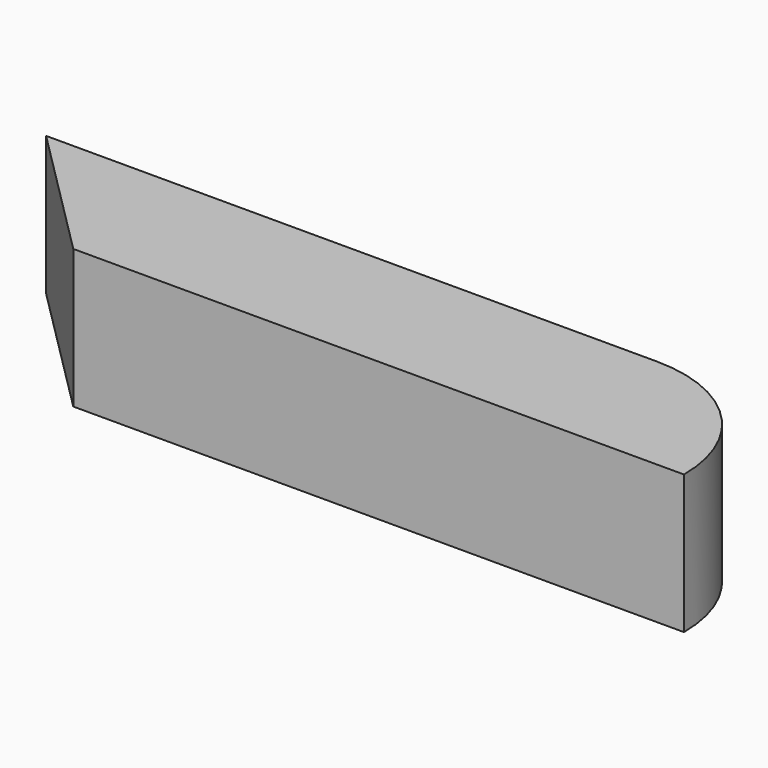
from build123d import *

# Parameters (mm, degrees)
F0_W     = 68.326
F0_H     = 12.446
F1_DEPTH = 12.7
F2_SIZE  = 12.44599
F3_R     = 12.44599
F5_D     = 6.35
F5_DEPTH = 8.89
F5_TIP   = 1.9077324654


# Not quite as in the source:
# - a fillet or chamfer is up to 0.001 mm smaller than in the source, because OpenCascade refuses the exact size


with BuildPart() as f1:
    # F0 (on Top) → F1 (new body)
    with BuildSketch(Plane.XY):
        Rectangle(F0_W, F0_H)
    extrude(amount=F1_DEPTH)

    # F2 (size 12.446 in the source; OpenCascade refuses exactly that, so slightly less here)
    f2_edges = [f1.edges().sort_by_distance(p)[0] for p in [
        (-34.163, -6.223, 6.35),
    ]]
    chamfer(f2_edges, length=F2_SIZE)

    # F3 (radius 12.446 in the source; OpenCascade refuses exactly that, so slightly less here)
    f3_edges = [f1.edges().sort_by_distance(p)[0] for p in [
        (34.163, 6.223, 6.35),
    ]]
    fillet(f3_edges, radius=F3_R)

    # F5
    with Locations(Plane(origin=(0, 0, 0), x_dir=(1, 0, 0), z_dir=(0, 0, -1))):
        with Locations((0, 0)):
            Hole(F5_D / 2, depth=F5_DEPTH)
            with Locations((0, 0, -(F5_DEPTH + F5_TIP / 2))):  # 118° drill point
                Cone(0, F5_D / 2, F5_TIP, mode=Mode.SUBTRACT)


solid = f1.part
